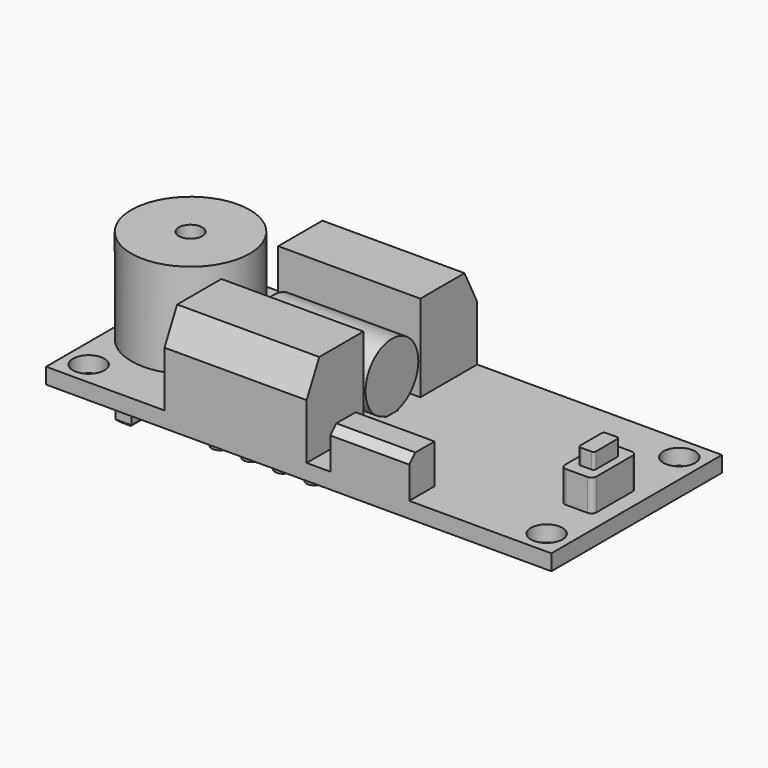
from build123d import *

# Parameters (mm, degrees)
F0_W      = 50.8
F0_H      = 21.43125
F1_DEPTH  = 1.5875
F2_R      = 1.5875
F3_DEPTH  = 3.175
F5_DEPTH  = 2.38125
F6_W      = 1.5875
F6_H      = 2.38125
F6_W_2    = 5.55625
F6_H_2    = 3.96875
F6_W_3    = 2.38125
F6_H_3    = 3.175
F6_W_4    = 6.35
F6_H_4    = 4.7625
F7_DEPTH  = 1.5875
F8_SIZE   = 0.254
F9_W      = 5.55625
F9_H      = 7.14375
F10_DEPTH = 2.38125
F11_SIZE  = 0.762
F12_SIZE  = 0.254
F13_R     = 5.953125
F14_DEPTH = 9.525
F15_R     = 1.190625
F16_DEPTH = 3.175
F17_W     = 14.2875
F17_H     = 7.14375
F18_DEPTH = 8.73125
F20_DEPTH = 15.24
F22_DEPTH = 11.90625
F23_W     = 3.175
F23_H     = 5.55625
F24_DEPTH = 3.175
F25_W     = 1.5875
F25_H     = 3.175
F26_DEPTH = 1.5875
F27_R     = 0.254
F28_R     = 0.508
F29_W     = 7.9375
F29_H     = 3.175
F30_DEPTH = 3.96875
F31_SIZE  = 0.762


# Not quite as in the source:
# - a length typed as a fraction of an inch, garbled in the dataset ("3 / 203.2 mm" for 3/8 in), is restored


with BuildPart() as f1:
    # F0 (on Top) → F1 (new body)
    with BuildSketch(Plane.XY):
        with Locations((2.7589667588, 1.3157454271)):
            Rectangle(F0_W, F0_H)
    extrude(amount=F1_DEPTH)

    # F2 (on face) → F3 (cut)
    with BuildSketch(Plane.XY.offset(1.5875)):
        with Locations((25.7777167588, -7.0186295729)):
            Circle(F2_R)
        with Locations((25.7777167588, 9.6501204271)):
            Circle(F2_R)
        with Locations((-20.2597832412, 9.6501204271)):
            Circle(F2_R)
        with Locations((-20.2597832412, -7.0186295729)):
            Circle(F2_R)
    extrude(amount=-F3_DEPTH, mode=Mode.SUBTRACT)

    # F4 (on face) → F5 (join)
    with BuildSketch(Plane(origin=(0, 0, 0), x_dir=(1, 0, 0), z_dir=(0, 0, -1))):
        with BuildLine():
            ThreePointArc((-5.1785332412, 6.2248795729), (-5.9722832412, 5.4311295706), (-5.1785332365, 4.6373795729))
            ThreePointArc((-5.1785332365, 4.6373795729), (-4.6172672319, 4.869863567), (-4.3847832412, 5.4311295729))
            ThreePointArc((-4.3847832412, 5.4311295729), (-4.6172672336, 5.9923955805), (-5.1785332412, 6.2248795729))
        make_face()
        with BuildLine():
            ThreePointArc((-2.0035332412, 6.2248795729), (-2.7972832412, 5.4311295729), (-2.0035332412, 4.6373795729))
            ThreePointArc((-2.0035332412, 4.6373795729), (-1.4422672336, 4.8698635653), (-1.2097832412, 5.4311295729))
            ThreePointArc((-1.2097832412, 5.4311295729), (-1.4422672336, 5.9923955805), (-2.0035332412, 6.2248795729))
        make_face()
        with BuildLine():
            ThreePointArc((1.1714667642, 6.2248795729), (0.3777167588, 5.4311295756), (1.1714667588, 4.6373795729))
            ThreePointArc((1.1714667588, 4.6373795729), (1.7327327664, 4.8698635653), (1.9652167588, 5.4311295729))
            ThreePointArc((1.9652167588, 5.4311295729), (1.7327327683, 5.9923955786), (1.1714667642, 6.2248795729))
        make_face()
        with BuildLine():
            ThreePointArc((-7.5597832412, -7.2688704271), (-7.7922672352, -6.7076044179), (-8.3535332458, -6.4751204271))
            ThreePointArc((-8.3535332458, -6.4751204271), (-9.1472832412, -7.2688704294), (-8.3535332412, -8.0626204271))
            ThreePointArc((-8.3535332412, -8.0626204271), (-7.7922672336, -7.8301364347), (-7.5597832412, -7.2688704271))
        make_face()
        with BuildLine():
            ThreePointArc((-4.3085832412, -7.2688704271), (-4.5410672352, -6.7076044179), (-5.1023332458, -6.4751204271))
            ThreePointArc((-5.1023332458, -6.4751204271), (-5.8960832412, -7.2688704294), (-5.1023332412, -8.0626204271))
            ThreePointArc((-5.1023332412, -8.0626204271), (-4.5410672336, -7.8301364347), (-4.3085832412, -7.2688704271))
        make_face()
        with BuildLine():
            ThreePointArc((-1.0573832412, -7.2688704271), (-1.2898672338, -6.7076044193), (-1.8511332418, -6.4751204271))
            ThreePointArc((-1.8511332418, -6.4751204271), (-2.6448832412, -7.2688704205), (-1.8511332549, -8.0626204271))
            ThreePointArc((-1.8511332549, -8.0626204271), (-1.2898672385, -7.8301364395), (-1.0573832412, -7.2688704271))
        make_face()
        with BuildLine():
            ThreePointArc((2.1938167588, -7.2688704271), (1.9613327658, -6.7076044189), (1.4000667571, -6.4751204271))
            ThreePointArc((1.4000667571, -6.4751204271), (0.6063167588, -7.2688704213), (1.4000667456, -8.0626204271))
            ThreePointArc((1.4000667456, -8.0626204271), (1.9613327617, -7.8301364393), (2.1938167588, -7.2688704271))
        make_face()
        with BuildLine():
            ThreePointArc((-8.3535332412, 6.2248795729), (-9.1472832412, 5.4311295729), (-8.3535332412, 4.6373795729))
            ThreePointArc((-8.3535332412, 4.6373795729), (-7.7922672336, 4.8698635653), (-7.5597832412, 5.4311295729))
            ThreePointArc((-7.5597832412, 5.4311295729), (-7.7922672336, 5.9923955805), (-8.3535332412, 6.2248795729))
        make_face()
    extrude(amount=F5_DEPTH)

    # F6 (on face) → F7 (join)
    with BuildSketch(Plane(origin=(0, 0, 0), x_dir=(1, 0, 0), z_dir=(0, 0, -1))):
        with Locations((-15.4972832412, 7.4155045729)):
            Rectangle(F6_W, F6_H)
        with Locations((-15.4972832412, 4.2405045729)):
            Rectangle(F6_W, F6_H)
        with Locations((-13.9097832412, -8.4594954271)):
            Rectangle(F6_W, F6_H)
        with Locations((-6.3691582412, 1.0655045729)):
            Rectangle(F6_W_2, F6_H_2)
        with Locations((0.7745917588, -0.1251204271)):
            Rectangle(F6_W_3, F6_H_3)
        with Locations((18.6339667588, 1.4623795729)):
            Rectangle(F6_W_4, F6_H_4)
        with Locations((18.2370917588, -4.8876204271)):
            Rectangle(F6_W_3, F6_H_4)
    extrude(amount=F7_DEPTH)

    # F8
    f8_edges = [f1.edges().sort_by_distance(p)[0] for p in [
        (-13.909783, 7.26887, -1.5875),
        (-14.703533, 8.459495, -1.5875),
        (-13.909783, 9.65012, -1.5875),
        (-13.116033, 8.459495, -1.5875),
        (-15.497283, -5.43113, -1.5875),
        (-16.291033, -4.240505, -1.5875),
        (-15.497283, -3.04988, -1.5875),
        (-14.703533, -4.240505, -1.5875),
        (-15.497283, -8.60613, -1.5875),
        (-16.291033, -7.415505, -1.5875),
        (-15.497283, -6.22488, -1.5875),
        (-14.703533, -7.415505, -1.5875),
        (-3.591033, -1.065505, -1.5875),
        (-6.369158, -3.04988, -1.5875),
        (-9.147283, -1.065505, -1.5875),
        (-6.369158, 0.91887, -1.5875),
        (0.774592, 1.71262, -1.5875),
        (1.965217, 0.12512, -1.5875),
        (0.774592, -1.46238, -1.5875),
        (-0.416033, 0.12512, -1.5875),
        (18.633967, 0.91887, -1.5875),
        (21.808967, -1.46238, -1.5875),
        (18.633967, -3.84363, -1.5875),
        (15.458967, -1.46238, -1.5875),
        (18.237092, 2.50637, -1.5875),
        (17.046467, 4.88762, -1.5875),
        (18.237092, 7.26887, -1.5875),
        (19.427717, 4.88762, -1.5875),
    ]]
    chamfer(f8_edges, length=F8_SIZE)

    # F9 (on face) → F10 (join)
    with BuildSketch(Plane(origin=(0, 0, 0), x_dir=(1, 0, 0), z_dir=(0, 0, -1))):
        with Locations((7.9183417588, -2.1094954271)):
            Rectangle(F9_W, F9_H)
    extrude(amount=F10_DEPTH)

    # F11
    f11_edges = [f1.edges().sort_by_distance(p)[0] for p in [
        (10.696467, 2.109495, -2.38125),
        (5.140217, 2.109495, -2.38125),
    ]]
    chamfer(f11_edges, length=F11_SIZE)

    # F12
    f12_edges = [f1.edges().sort_by_distance(p)[0] for p in [
        (7.918342, -1.46238, -2.38125),
        (7.918342, 5.68137, -2.38125),
    ]]
    chamfer(f12_edges, length=F12_SIZE)

    # F13 (on face) → F14 (join)
    with BuildSketch(Plane.XY.offset(1.5875)):
        with Locations((-16.6879082412, 1.3157454271)):
            Circle(F13_R)
    extrude(amount=F14_DEPTH)

    # F15 (on face) → F16 (cut)
    with BuildSketch(Plane.XY.offset(11.1125)):
        with Locations((-16.6879082412, 1.3157454271)):
            Circle(F15_R)
    extrude(amount=-F16_DEPTH, mode=Mode.SUBTRACT)

    # F17 (on face) → F18 (join)
    with BuildSketch(Plane.XY.offset(1.5875)):
        with Locations((-3.5910332412, 8.4594954271)):
            Rectangle(F17_W, F17_H)
        with Locations((-3.5910332412, -5.8280045729)):
            Rectangle(F17_W, F17_H)
    extrude(amount=F18_DEPTH)

    # F19 (on face) → F20 (cut)
    with BuildSketch(Plane.YZ.offset(3.5527167588)):
        Polygon((-12.6245096326, 12.3970924459), (-9.3998795729, 7.14375), (-7.8123795729, 10.31875), (-6.8544447422, 13.4305364035), align=None)
        Polygon((11.735675374, 13.160722746), (10.4438704271, 10.31875), (12.0313704271, 7.14375), (15.6484242786, 9.6412404954), (16.4722963069, 13.6774447247), align=None)
    extrude(amount=-F20_DEPTH, mode=Mode.SUBTRACT)

    # F21 (on face) → F22 (join)
    with BuildSketch(Plane.YZ.offset(3.5527167588)):
        with BuildLine():
            ThreePointArc((2.0925854259, 1.6797255876), (3.9220601171, 2.8522266244), (4.6336204271, 4.905375))
            ThreePointArc((4.6336204271, 4.905375), (-0.7374029485, 7.51168969), (0.5389054283, 1.6797255876))
            Line((0.5389054283, 1.6797255876), (2.0925854259, 1.6797255876))
        make_face()
        with BuildLine():
            Line((2.0925854259, 1.6797255876), (0.5389054283, 1.6797255876))
            ThreePointArc((0.5389054283, 1.6797255876), (1.3157454271, 1.5875), (2.0925854259, 1.6797255876))
        make_face()
        with BuildLine():
            ThreePointArc((2.0925854259, 1.6797255876), (1.3157454271, 1.5875), (0.5389054283, 1.6797255876))
            Line((0.5389054283, 1.6797255876), (0.5389054283, 1.5345554566))
            Line((0.5389054283, 1.5345554566), (2.0925854259, 1.5345554566))
            Line((2.0925854259, 1.5345554566), (2.0925854259, 1.6797255876))
        make_face()
    extrude(amount=-F22_DEPTH)

    # F23 (on face) → F24 (join)
    with BuildSketch(Plane.XY.offset(1.5875)):
        with Locations((24.9839667588, 0.5219954271)):
            Rectangle(F23_W, F23_H)
    extrude(amount=F24_DEPTH)

    # F25 (on face) → F26 (join)
    with BuildSketch(Plane.XY.offset(4.7625)):
        with Locations((24.9839667588, 0.5219954271)):
            Rectangle(F25_W, F25_H)
    extrude(amount=F26_DEPTH)

    # F27
    f27_edges = [f1.edges().sort_by_distance(p)[0] for p in [
        (25.777717, -1.065505, 5.55625),
        (24.190217, -1.065505, 5.55625),
        (24.190217, 2.109495, 5.55625),
        (25.777717, 2.109495, 5.55625),
    ]]
    fillet(f27_edges, radius=F27_R)

    # F28
    f28_edges = [f1.edges().sort_by_distance(p)[0] for p in [
        (26.571467, 3.30012, 3.175),
        (23.396467, 3.30012, 3.175),
        (26.571467, -2.25613, 3.175),
        (23.396467, -2.25613, 3.175),
    ]]
    fillet(f28_edges, radius=F28_R)

    # F29 (on face) → F30 (join)
    with BuildSketch(Plane.XY.offset(1.5875)):
        with Locations((9.9027167588, -7.8123795729)):
            Rectangle(F29_W, F29_H)
    extrude(amount=F30_DEPTH)

    # F31
    f31_edges = [f1.edges().sort_by_distance(p)[0] for p in [
        (9.902717, -9.39988, 5.55625),
    ]]
    chamfer(f31_edges, length=F31_SIZE)


solid = f1.part
